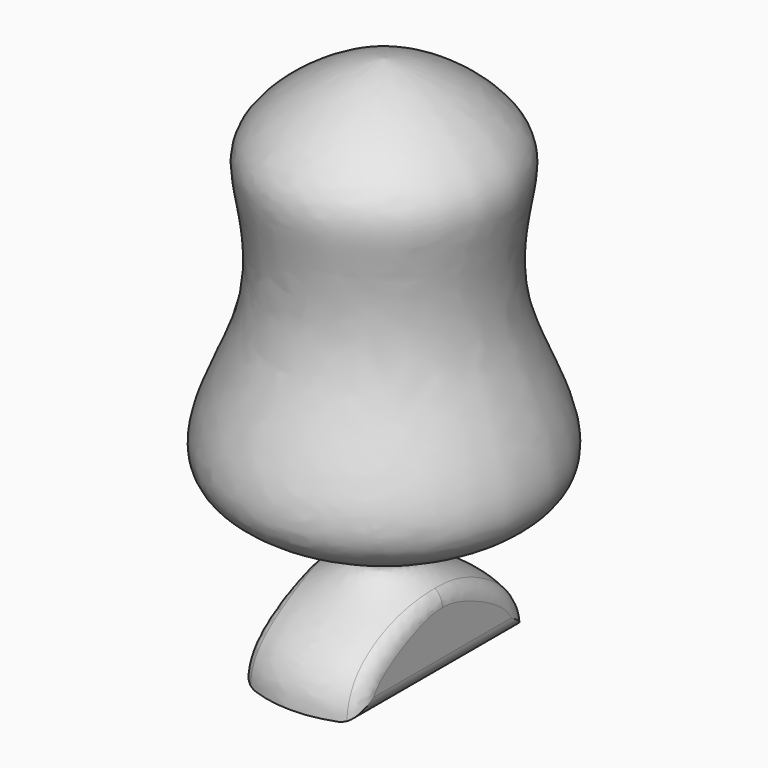
from build123d import *

# Parameters (mm, degrees)
F3_DEPTH = 15.0184705853
F4_R     = 3


with BuildPart() as f1:
    # F0 (on Front) → F1 (revolve)
    with BuildSketch(Plane.XZ):
        with BuildLine():
            Line((0, 90), (0, 0))
            Line((0, 0), (20, 0))
            add(Edge.make_bspline(
                [(0, 90), (6.9209166377, 89.4050945379), (21.651667386, 80.2388254358), (20.0001646985, 69.8224346963), (16.4655149949, 50.9816762749), (35.256642876, 24.9263157542), (-0.4699743666, 18.4653741452), (12.6406494502, 10.658477606), (19.962757975, 5.6484302204), (20, 0)],
                knots=[0, 0, 0, 0, 0.1658980907, 0.2728118869, 0.4279863224, 0.6005308183, 0.7666707323, 0.8668712718, 1, 1, 1, 1], degree=3))
        make_face()
    revolve(axis=Axis((0, 0, 45), (0, 0, 1)))

    # F2 (on face) → F3 (cut)
    with BuildSketch(Plane(origin=(0, 0, 0), x_dir=(1, 0, 0), z_dir=(0, 0, -1))):
        with BuildLine():
            Line((-10, -17.3205080757), (-10, 17.3205080757))
            ThreePointArc((-10, 17.3205080757), (-20, 0), (-10, -17.3205080757))
        make_face()
        with BuildLine():
            ThreePointArc((20, 0), (17.3205080757, 10), (10, 17.3205080757))
            Line((10, 17.3205080757), (10, -17.3205080757))
            ThreePointArc((10, -17.3205080757), (17.3205080757, -10), (20, 0))
        make_face()
    extrude(amount=-F3_DEPTH, mode=Mode.SUBTRACT)

    # F4
    f4_edges = [f1.edges().sort_by_distance(p)[0] for p in [
        (-10, 0, 12.167863),
        (10, -10.978539, 8.951115),
        (10, 10.978539, 8.951115),
        (-10, 0, 0),
        (10, 0, 0),
    ]]
    fillet(f4_edges, radius=F4_R)


solid = f1.part
